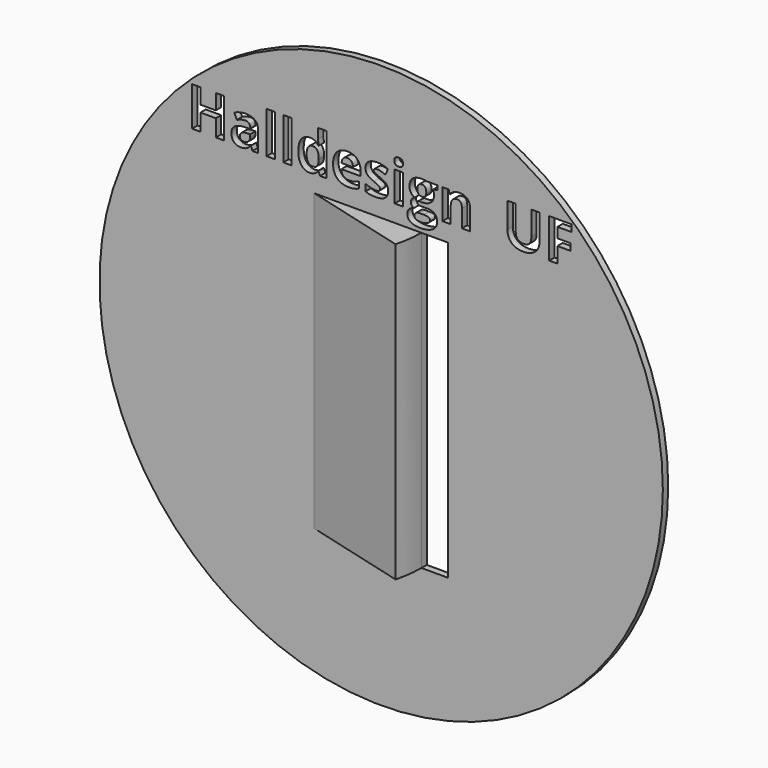
from build123d import *

# Parameters (mm, degrees)
F0_W         = 40
F0_H         = 110
F1_DEPTH     = 2.5
F0_R         = 105
F2_DEPTH     = 2.5
F3_W         = 40
F3_H         = 110
F4_ANGLE     = 15
F5_TEXT_SIZE = 20.4737128783
F7_DEPTH     = 50


# Not quite as in the source:
# - a feature names something its author has since deleted; it is built from what else it names
# - Text() gives the source's letters only with a copy of the font that has no kerning and outlines rounded to 1/6400 em; it was checked with that copy


with BuildPart() as f1:
    # F0 (on Front) → F1 (new body)
    with BuildSketch(Plane.XZ):
        with Locations((-61.7234227247, 37.4147482216)):
            Rectangle(F0_W, F0_H)
    extrude(amount=F1_DEPTH)


with BuildPart() as f2:
    # F0 (on Front) → F2 (new body)
    with BuildSketch(Plane.XZ):
        with Locations((-56.7234227247, 37.4147482216)):
            Circle(F0_R)
        Polygon((-81.7234227247, -17.5852517784), (-81.7234227247, 92.4147482216), (-41.7234227247, 92.4147482216), (-31.7234227247, 92.4147482216), (-31.7234227247, -17.5852517784), (-41.7234227247, -17.5852517784), align=None, mode=Mode.SUBTRACT)
    extrude(amount=F2_DEPTH)

    # F5 (on face) → F7 (cut)
    with BuildSketch(Plane.XZ.offset(2.5)):
        with Locations((-129.067607082, 98.774391041)):
            Text('Halldesign  UF', F5_TEXT_SIZE, font='Open Sans', font_style=FontStyle.BOLD, text_align=(TextAlign.LEFT, TextAlign.BOTTOM))
    extrude(amount=-F7_DEPTH, mode=Mode.SUBTRACT)


with BuildPart() as f4:
    # F3 (on face) → F4 (revolve)
    with BuildSketch(Plane.XZ.offset(2.5)):
        with Locations((-61.7234227247, 37.4147482216)):
            Rectangle(F3_W, F3_H)
    revolve(axis=Axis((-81.7234227247, -2.5, 20.3633494675), (0, 0, -1)), revolution_arc=F4_ANGLE)


solid = Compound([f1.part, f2.part, f4.part])
